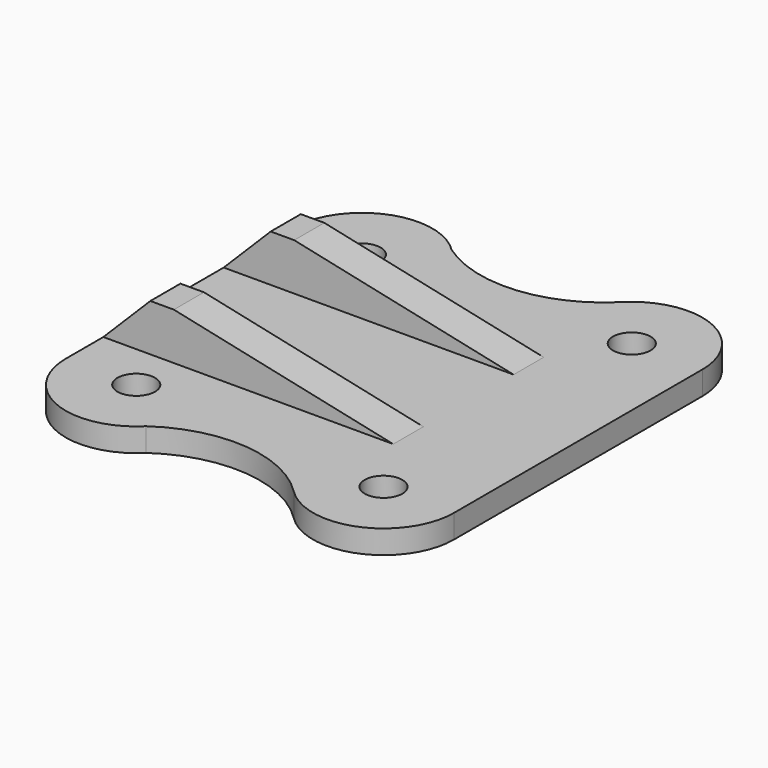
from build123d import *

# Parameters (mm, degrees)
F1_DEPTH    = 5
F2_R        = 4
F3_DEPTH    = 25
F5_W        = 85
F5_H        = 8
F6_DEPTH    = 15
F7_T4_DEPTH = 371.701063592
F7_T9_DEPTH = 371.701063592
F8_SIZE     = 10


# Not quite as in the source:
# - a fillet or chamfer that OpenCascade refuses, or shapes differently, is made with other operations: its cross-section is extruded or revolved along the edge and cut away or added
# - a feature names something its author has since deleted; it is built from what else it names


with BuildPart() as f1:
    # F0 (on Top) → F1 (new body)
    with BuildSketch(Plane.XY):
        with BuildLine():
            ThreePointArc((-19.3933982822, 40.6066017178), (-16.1418070123, 35.7402514855), (-15, 30))
            ThreePointArc((-15, 30), (-30, 15), (-45, 30))
            Line((-45, 30), (-45, -30))
            ThreePointArc((-45, -30), (-30, -15), (-15, -30))
            ThreePointArc((-15, -30), (-16.1418070123, -35.7402514855), (-19.3933982822, -40.6066017178))
            ThreePointArc((-19.3933982822, -40.6066017178), (-1.9551429216, -35.9702766297), (14.3933982822, -43.6066017178))
            ThreePointArc((14.3933982822, -43.6066017178), (19.2597485145, -19.1418070123), (40, -33))
            Line((40, -33), (40, 33))
            ThreePointArc((40, 33), (19.2597485145, 19.1418070123), (14.3933982822, 43.6066017178))
            ThreePointArc((14.3933982822, 43.6066017178), (-1.9551429216, 35.9702766297), (-19.3933982822, 40.6066017178))
        make_face()
        with BuildLine():
            ThreePointArc((-15, -30), (-30, -15), (-45, -30))
            ThreePointArc((-45, -30), (-35.7402514855, -43.8581929877), (-19.3933982822, -40.6066017178))
            ThreePointArc((-19.3933982822, -40.6066017178), (-16.1418070123, -35.7402514855), (-15, -30))
        make_face()
        with BuildLine():
            ThreePointArc((-45, 30), (-30, 15), (-15, 30))
            ThreePointArc((-15, 30), (-16.1418070123, 35.7402514855), (-19.3933982822, 40.6066017178))
            ThreePointArc((-19.3933982822, 40.6066017178), (-35.7402514855, 43.8581929877), (-45, 30))
        make_face()
        with BuildLine():
            ThreePointArc((40, 33), (30.7402514855, 46.8581929877), (14.3933982822, 43.6066017178))
            ThreePointArc((14.3933982822, 43.6066017178), (19.2597485145, 19.1418070123), (40, 33))
        make_face()
        with BuildLine():
            ThreePointArc((14.3933982822, -43.6066017178), (30.7402514855, -46.8581929877), (40, -33))
            ThreePointArc((40, -33), (19.2597485145, -19.1418070123), (14.3933982822, -43.6066017178))
        make_face()
    extrude(amount=F1_DEPTH)


with BuildPart() as f3:
    # F2 (on Top) → F3 (new body)
    with BuildSketch(Plane.XY):
        with Locations((-30, 30)):
            Circle(F2_R)
    extrude(amount=F3_DEPTH)


with BuildPart() as f3b:
    # F2 (on Top) → F3, piece 2 (new body)
    with BuildSketch(Plane.XY):
        with Locations((25, 33)):
            Circle(F2_R)
    extrude(amount=F3_DEPTH)


with BuildPart() as f3c:
    # F2 (on Top) → F3, piece 3 (new body)
    with BuildSketch(Plane.XY):
        with Locations((25, -33)):
            Circle(F2_R)
    extrude(amount=F3_DEPTH)


with BuildPart() as f3d:
    # F2 (on Top) → F3, piece 4 (new body)
    with BuildSketch(Plane.XY):
        with Locations((-30, -30)):
            Circle(F2_R)
    extrude(amount=F3_DEPTH)


with BuildPart() as f1_1:
    add(f1.part)

    # F4: cut F3, F3b, F3c, F3d
    add(f3.part, mode=Mode.SUBTRACT)
    add(f3b.part, mode=Mode.SUBTRACT)
    add(f3c.part, mode=Mode.SUBTRACT)
    add(f3d.part, mode=Mode.SUBTRACT)

    # F5 (on Top) → F6 (join)
    with BuildSketch(Plane.XY):
        with Locations((-2.5, 16)):
            Rectangle(F5_W, F5_H)
        with Locations((-2.5, -16)):
            Rectangle(F5_W, F5_H)
    extrude(amount=F6_DEPTH)

    # F7: chamfer of 15 x 70 on 2 edges, made by hand


with BuildPart() as f7_tool2:
    # F7_s3 → F7_t4 (new body)
    with BuildSketch(Plane.XZ.offset(169.850531796)):
        Polygon((-30, 15), (40, 0), (40, 15), align=None)
    extrude(amount=-F7_T4_DEPTH)

    split(bisect_by=Plane.XY.offset(5), keep=Keep.TOP)


with BuildPart() as f1_2:
    add(f1_1.part)

    # F7_t1: cut F7_tool2
    add(f7_tool2.part, mode=Mode.SUBTRACT)


with BuildPart() as f7_tool7:
    # F7_s8 → F7_t9 (new body)
    with BuildSketch(Plane.XZ.offset(201.850531796)):
        Polygon((-30, 15), (40, 0), (40, 15), align=None)
    extrude(amount=-F7_T9_DEPTH)

    split(bisect_by=Plane.XY.offset(5), keep=Keep.TOP)


with BuildPart() as f1_3:
    add(f1_2.part)

    # F7_t6: cut F7_tool7
    add(f7_tool7.part, mode=Mode.SUBTRACT)

    # F8
    f8_edges = [f1_3.edges().sort_by_distance(p)[0] for p in [
        (-45, 16, 15),
        (-45, -16, 15),
    ]]
    chamfer(f8_edges, length=F8_SIZE)


solid = f1_3.part
